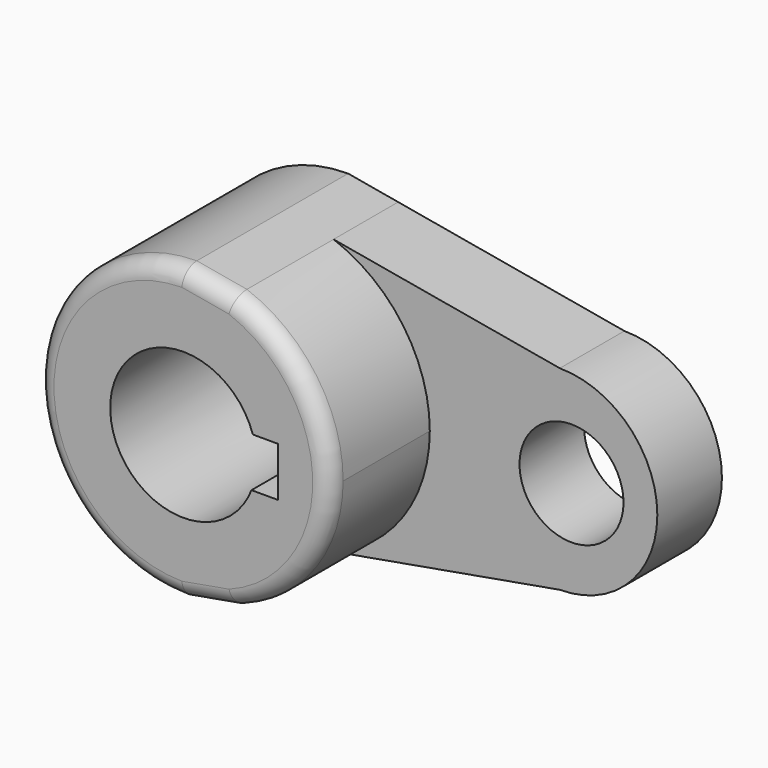
from build123d import *

# Parameters (mm, degrees)
F1_DEPTH    = 15.7734
F3_DEPTH    = 24.4602
F4_T1_DEPTH = 37.9988318329
F4_T3_DEPTH = 37.9988318329
F4_T6_ANGLE = 213.1574660215
F4_T8_ANGLE = 173.1044855741
F6_DEPTH    = 40.2346
F7_R        = 10.16
F8_DEPTH    = 15.7744


# Not quite as in the source:
# - a fillet or chamfer that OpenCascade refuses, or shapes differently, is made with other operations: its cross-section is extruded or revolved along the edge and cut away or added


with BuildPart() as f1:
    # F0 (on Front) → F1 (new body)
    with BuildSketch(Plane.XZ):
        with BuildLine():
            Line((53.975, 19.05), (9.780704698, 26.8489932886))
            Line((9.780704698, 26.8489932886), (0, 28.575))
            ThreePointArc((0, 28.575), (-28.575, 0), (0, -28.575))
            Line((0, -28.575), (9.780704698, -26.8489932886))
            Line((9.780704698, -26.8489932886), (53.975, -19.05))
            ThreePointArc((53.975, -19.05), (73.025, 0), (53.975, 19.05))
        make_face()
    extrude(amount=-F1_DEPTH)

    # F2 (on face) → F3 (join)
    with BuildSketch(Plane.XZ):
        with BuildLine():
            Line((9.780704698, 26.8489932886), (0, 28.575))
            ThreePointArc((0, 28.575), (-28.575, 0), (0, -28.575))
            Line((0, -28.575), (9.780704698, -26.8489932886))
            ThreePointArc((9.780704698, -26.8489932886), (23.4095521288, -16.3866864902), (28.575, 0))
            ThreePointArc((28.575, 0), (23.4095521288, 16.3866864902), (9.780704698, 26.8489932886))
        make_face()
    extrude(amount=F3_DEPTH)

    # F4: fillet of radius 3.302 on 4 edges, made by hand

    # F4_s2 → F4_t1 (cut)
    with BuildSketch(Plane(origin=(-18.7103124217, 0, -3.3018198391), x_dir=(0, 1, 0), z_dir=(0.9847835588, 0, 0.1737853339))):
        with BuildLine():
            ThreePointArc((-21.1582, -28.1401901932), (-23.4930665915, -27.1730567847), (-24.4602, -24.8381901932))
            Line((-24.4602, -24.8381901932), (-24.4602, -28.1401901932))
            Line((-24.4602, -28.1401901932), (-21.1582, -28.1401901932))
        make_face()
    extrude(amount=F4_T1_DEPTH, mode=Mode.SUBTRACT)

    # F4_s4 → F4_t3 (cut)
    with BuildSketch(Plane(origin=(18.7103124217, 0, -3.3018198391), x_dir=(0, 1, 0), z_dir=(-0.9847835588, 0, 0.1737853339))):
        with BuildLine():
            ThreePointArc((-21.1582, -28.1401901932), (-23.4930665915, -27.1730567847), (-24.4602, -24.8381901932))
            Line((-24.4602, -24.8381901932), (-24.4602, -28.1401901932))
            Line((-24.4602, -28.1401901932), (-21.1582, -28.1401901932))
        make_face()
    extrude(amount=F4_T3_DEPTH, mode=Mode.SUBTRACT)

    # F4_s5 → F4_t6 (revolve, cut)
    with BuildSketch(Plane(origin=(0, 0, 0), x_dir=(0, 1, 0), z_dir=(0.95842855, 0, -0.2853326385))):
        with BuildLine():
            ThreePointArc((-24.4602, 25.273), (-23.4930665915, 27.6078665915), (-21.1582, 28.575))
            Line((-21.1582, 28.575), (-24.4602, 28.575))
            Line((-24.4602, 28.575), (-24.4602, 25.273))
        make_face()
    revolve(axis=Axis((0, -24.4602, 0), (0, -1, 0)), revolution_arc=F4_T6_ANGLE, mode=Mode.SUBTRACT)

    # F4_s7 → F4_t8 (revolve, cut)
    with BuildSketch(Plane(origin=(0, 0, 0), x_dir=(0, 1, 0), z_dir=(-0.9981900481, 0, 0.0601384063))):
        with BuildLine():
            ThreePointArc((-21.1582, -28.575), (-23.4930665915, -27.6078665915), (-24.4602, -25.273))
            Line((-24.4602, -25.273), (-24.4602, -28.575))
            Line((-24.4602, -28.575), (-21.1582, -28.575))
        make_face()
    revolve(axis=Axis((0, -24.4602, 0), (0, 1, 0)), revolution_arc=F4_T8_ANGLE, mode=Mode.SUBTRACT)

    # F5 (on face) → F6 (cut, through all)
    with BuildSketch(Plane.XZ.offset(24.4602)):
        with BuildLine():
            Line((18.5293, 4.4565453057), (13.574677167, 4.4565453057))
            ThreePointArc((13.574677167, 4.4565453057), (-14.2821064756, 0.3925440984), (13.3093916754, -5.1954546943))
            Line((13.3093916754, -5.1954546943), (18.5293, -5.1954546943))
            Line((18.5293, -5.1954546943), (18.5293, 4.4565453057))
        make_face()
    extrude(amount=-F6_DEPTH, mode=Mode.SUBTRACT)

    # F7 (on face) → F8 (cut, through all)
    with BuildSketch(Plane.XZ):
        with Locations((56.261, 0)):
            Circle(F7_R)
    extrude(amount=-F8_DEPTH, mode=Mode.SUBTRACT)


solid = f1.part
